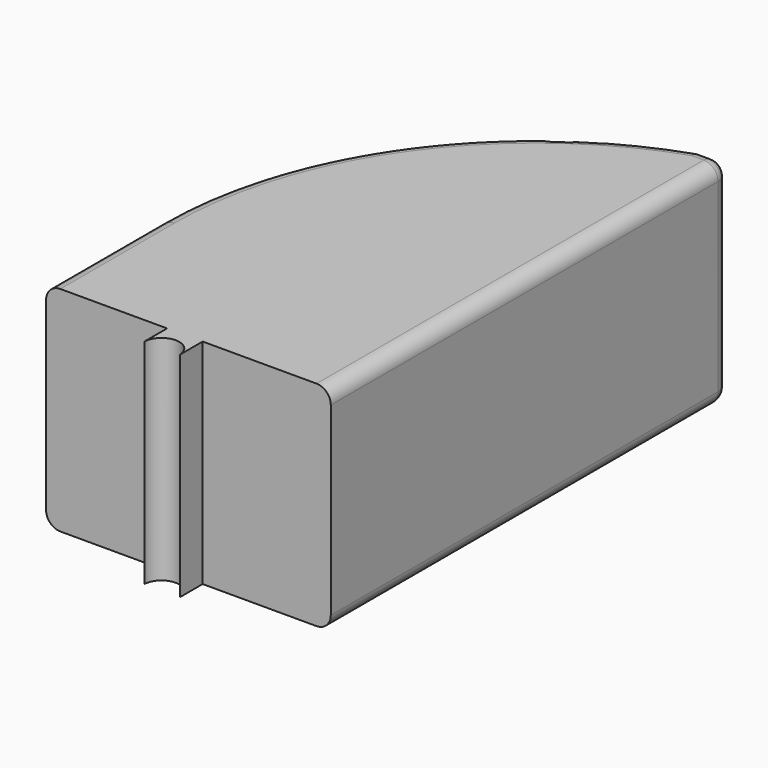
from build123d import *

# Parameters (mm, degrees)
F0_W         = 20
F0_H         = 15
F1_DEPTH     = 10
F2_R         = 1
F4_DEPTH     = 15
F5_T1_DEPTH  = 30
F5_T3_DEPTH  = 8.75
F5_T6_ANGLE  = 80.7474763736
F5_T8_ANGLE  = 80.7474763736
F6_R         = 1
F7_T1_DEPTH  = 13
F7_S5_W      = 1
F7_S5_H      = 1
F7_T6_DEPTH  = 1
F7_S11_W     = 1
F7_S11_H     = 1
F7_T12_DEPTH = 1
F9_DEPTH     = 15


# Not quite as in the source:
# - a fillet or chamfer that OpenCascade refuses, or shapes differently, is made with other operations: its cross-section is extruded or revolved along the edge and cut away or added


with BuildPart() as f1:
    # F0 (on Front) → F1 (new body)
    with BuildSketch(Plane.XZ):
        with Locations((-10, 7.5)):
            Rectangle(F0_W, F0_H)
    extrude(amount=F1_DEPTH)

    # F2
    f2_edges = [f1.edges().sort_by_distance(p)[0] for p in [
        (-20, -5, 15),
        (0, -5, 15),
        (-20, -5, 0),
        (0, -5, 0),
    ]]
    fillet(f2_edges, radius=F2_R)

    # F3 (on Top) → F4 (join)
    with BuildSketch(Plane.XY):
        with BuildLine():
            Line((-20, 0), (0, 0))
            Line((0, 0), (0, 25))
            Line((0, 25), (-2, 25))
            ThreePointArc((-2, 25), (-15.0318358344, 15.4029218007), (-20, 0))
        make_face()
    extrude(amount=F4_DEPTH)

    # F5: fillet of radius 1 on 6 edges, made by hand

    # F5_s2 → F5_t1 (cut)
    with BuildSketch(Plane.XZ.offset(-27.5)):
        with BuildLine():
            ThreePointArc((-1, 15), (-0.2928932188, 14.7071067812), (0, 14))
            Line((0, 14), (0, 15))
            Line((0, 15), (-1, 15))
        make_face()
        with BuildLine():
            ThreePointArc((-1, 0), (-0.2928932188, 0.2928932188), (0, 1))
            Line((0, 1), (0, 0))
            Line((0, 0), (-1, 0))
        make_face()
    extrude(amount=F5_T1_DEPTH, mode=Mode.SUBTRACT)

    # F5_s4 → F5_t3 (cut)
    with BuildSketch(Plane.YZ.offset(-6.25)):
        with BuildLine():
            ThreePointArc((25, 14), (24.7071067812, 14.7071067812), (24, 15))
            Line((24, 15), (25, 15))
            Line((25, 15), (25, 14))
        make_face()
        with BuildLine():
            ThreePointArc((25, 1), (24.7071067812, 0.2928932188), (24, 0))
            Line((24, 0), (25, 0))
            Line((25, 0), (25, 1))
        make_face()
    extrude(amount=F5_T3_DEPTH, mode=Mode.SUBTRACT)

    # F5_s5 → F5_t6 (revolve, cut)
    with BuildSketch(Plane(origin=(6.1966627118, 1.0094707841, 0), x_dir=(0, 0, 1), z_dir=(0.9869892856, 0.1607860383, 0))):
        with BuildLine():
            ThreePointArc((14, -25.3383332565), (14.7071067812, -25.0454400377), (15, -24.3383332565))
            Line((15, -24.3383332565), (15, -25.3383332565))
            Line((15, -25.3383332565), (14, -25.3383332565))
        make_face()
    revolve(axis=Axis((6.3611111111, 0, 15), (0, 0, 1)), revolution_arc=F5_T6_ANGLE, mode=Mode.SUBTRACT)

    # F5_s7 → F5_t8 (revolve, cut)
    with BuildSketch(Plane(origin=(6.1966627118, 1.0094707841, 0), x_dir=(0, 0, 1), z_dir=(0.9869892856, 0.1607860383, 0))):
        with BuildLine():
            ThreePointArc((1, -25.3383332565), (0.2928932188, -25.0454400377), (0, -24.3383332565))
            Line((0, -24.3383332565), (0, -25.3383332565))
            Line((0, -25.3383332565), (1, -25.3383332565))
        make_face()
    revolve(axis=Axis((6.3611111111, 0, 0), (0, 0, 1)), revolution_arc=F5_T8_ANGLE, mode=Mode.SUBTRACT)

    # F6
    f6_edges = [f1.edges().sort_by_distance(p)[0] for p in [
        (-2, 25, 7.5),
    ]]
    fillet(f6_edges, radius=F6_R)

    # F7: fillet of radius 1 on 1 edges, made by hand

    # F7_s2 → F7_t1 (cut)
    with BuildSketch(Plane.XY.offset(1)):
        with BuildLine():
            ThreePointArc((-1, 25), (-0.2928932188, 24.7071067812), (0, 24))
            Line((0, 24), (0, 25))
            Line((0, 25), (-1, 25))
        make_face()
    extrude(amount=F7_T1_DEPTH, mode=Mode.SUBTRACT)


with BuildPart() as f7_tool4:
    # F7_s5 → F7_t6 (new body)
    with BuildSketch(Plane.XZ.offset(-24)):
        with Locations((-0.5, 0.5)):
            Rectangle(F7_S5_W, F7_S5_H)
    extrude(amount=-F7_T6_DEPTH)

    # F7_s7 → F7_t8 (revolve, cut)
    with BuildSketch(Plane(origin=(-1, 24, 1), x_dir=(-0.7071067812, 0, 0.7071067812), z_dir=(-0.7071067812, 0, -0.7071067812))):
        with BuildLine():
            ThreePointArc((0, -1), (1, 0), (0, 1))
            Line((0, 1), (0, -1))
        make_face()
    revolve(axis=Axis((-1, 24, 1), (0, 1, 0)), mode=Mode.SUBTRACT)


with BuildPart() as f1_1:
    add(f1.part)

    # F7_t3: cut F7_tool4
    add(f7_tool4.part, mode=Mode.SUBTRACT)


with BuildPart() as f7_tool10:
    # F7_s11 → F7_t12 (new body)
    with BuildSketch(Plane.XZ.offset(-24)):
        with Locations((-0.5, 14.5)):
            Rectangle(F7_S11_W, F7_S11_H)
    extrude(amount=-F7_T12_DEPTH)

    # F7_s13 → F7_t14 (revolve, cut)
    with BuildSketch(Plane(origin=(-1, 24, 14), x_dir=(-0.7071067812, 0, -0.7071067812), z_dir=(0.7071067812, 0, -0.7071067812))):
        with BuildLine():
            ThreePointArc((0, -1), (1, 0), (0, 1))
            Line((0, 1), (0, -1))
        make_face()
    revolve(axis=Axis((-1, 24, 14), (0, 1, 0)), mode=Mode.SUBTRACT)


with BuildPart() as f1_2:
    add(f1_1.part)

    # F7_t9: cut F7_tool10
    add(f7_tool10.part, mode=Mode.SUBTRACT)

    # F8 (on Top) → F9 (join, through all)
    with BuildSketch(Plane.XY):
        with BuildLine():
            Line((-9, -10), (-11.4979991994, -10))
            Line((-11.4979991994, -10), (-11.4979991994, -12))
            ThreePointArc((-11.4979991994, -12), (-10.2489995997, -10.8), (-9, -12))
            Line((-9, -12), (-9, -10))
        make_face()
    extrude(amount=F9_DEPTH)


solid = f1_2.part
